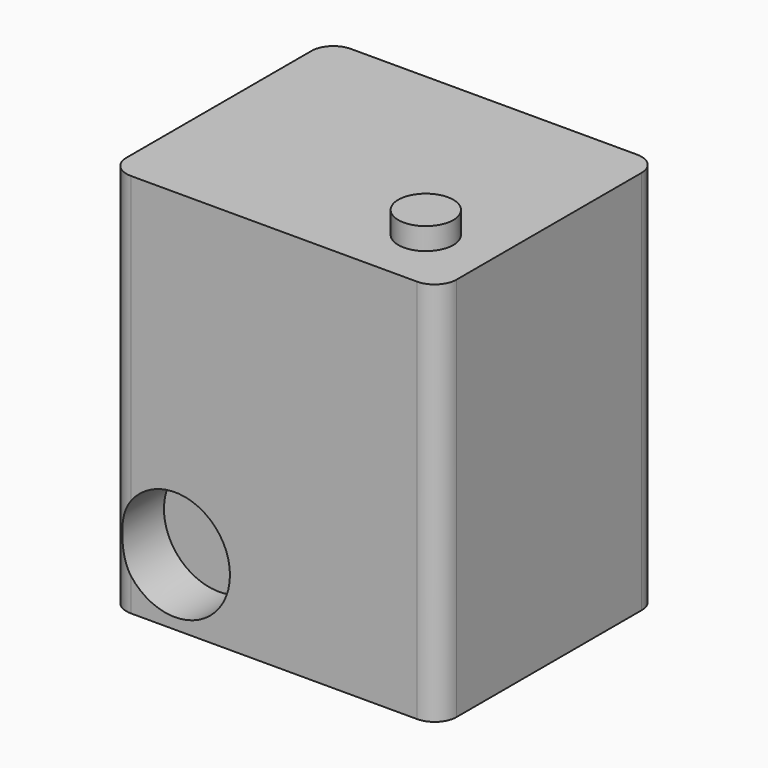
from build123d import *

# Parameters (mm, degrees)
F0_W        = 38.1
F0_H        = 44.45
F1_DEPTH    = 31.75
F2_R        = 6.35
F3_DEPTH    = 6.35
F4_R        = 3.175
F5_DEPTH    = 2.54
F6_T1_DEPTH = 57.15


# Not quite as in the source:
# - a fillet or chamfer that OpenCascade refuses, or shapes differently, is made with other operations: its cross-section is extruded or revolved along the edge and cut away or added


with BuildPart() as f1:
    # F0 (on Front) → F1 (new body)
    with BuildSketch(Plane.XZ):
        Rectangle(F0_W, F0_H)
    extrude(amount=F1_DEPTH)

    # F2 (on face) → F3 (cut)
    with BuildSketch(Plane.XZ.offset(31.75)):
        with Locations((-11.43, -14.605)):
            Circle(F2_R)
    extrude(amount=-F3_DEPTH, mode=Mode.SUBTRACT)

    # F4 (on face) → F5 (join)
    with BuildSketch(Plane.XY.offset(22.225)):
        with Locations((11.43, -24.13)):
            Circle(F4_R)
    extrude(amount=F5_DEPTH)

    # F6: fillet of radius 2.54 on 4 edges, made by hand

    # F6_s2 → F6_t1 (cut)
    with BuildSketch(Plane.XY.offset(-28.575)):
        with BuildLine():
            ThreePointArc((-16.51, -31.75), (-18.3060512242, -31.0060512242), (-19.05, -29.21))
            Line((-19.05, -29.21), (-19.05, -31.75))
            Line((-19.05, -31.75), (-16.51, -31.75))
        make_face()
        with BuildLine():
            ThreePointArc((19.05, -29.21), (18.3060512242, -31.0060512242), (16.51, -31.75))
            Line((16.51, -31.75), (19.05, -31.75))
            Line((19.05, -31.75), (19.05, -29.21))
        make_face()
        with BuildLine():
            ThreePointArc((-16.51, 0), (-18.3060512242, -0.7439487758), (-19.05, -2.54))
            Line((-19.05, -2.54), (-19.05, 0))
            Line((-19.05, 0), (-16.51, 0))
        make_face()
        with BuildLine():
            ThreePointArc((19.05, -2.54), (18.3060512242, -0.7439487758), (16.51, 0))
            Line((16.51, 0), (19.05, 0))
            Line((19.05, 0), (19.05, -2.54))
        make_face()
    extrude(amount=F6_T1_DEPTH, mode=Mode.SUBTRACT)


solid = f1.part
